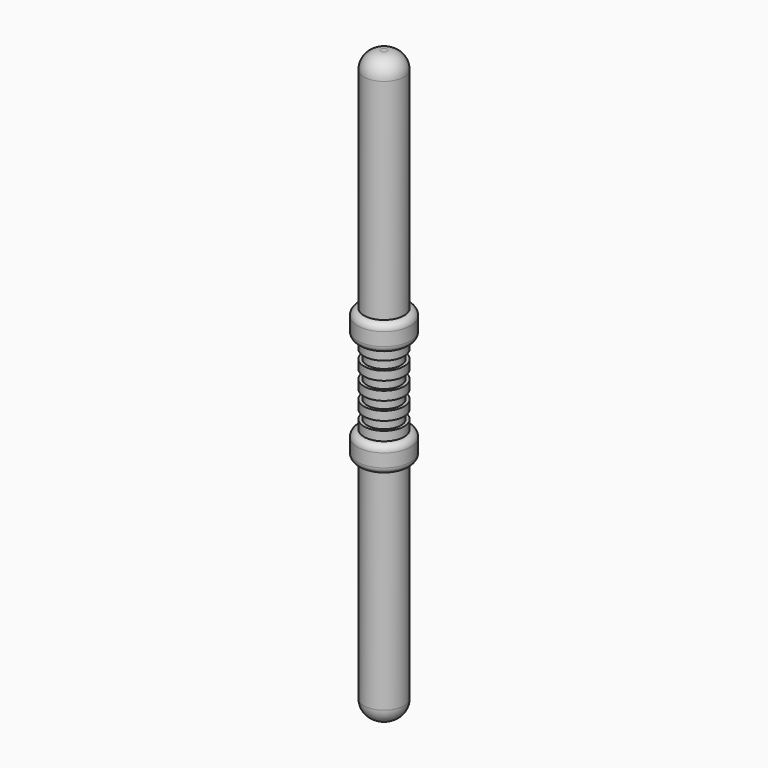
from build123d import *

# Parameters (mm, degrees)
F0_R          = 1.5
F1_DEPTH      = 3
F2_R          = 2
F3_DEPTH      = 2
F4_R          = 1.5
F5_DEPTH      = 17
F6_R          = 1.27
F8_W          = 0.5104065668
F8_H          = 0.6614452832
F10_S5_R      = 1.5
F10_T6_DEPTH  = 5
F10_S11_R     = 1.5
F10_T12_DEPTH = 5
F10_S17_R     = 1.5
F10_T18_DEPTH = 5
F10_S23_R     = 1.5
F10_T24_DEPTH = 5


# Not quite as in the source:
# - a fillet or chamfer that OpenCascade refuses, or shapes differently, is made with other operations: its cross-section is extruded or revolved along the edge and cut away or added


with BuildPart() as f1:
    # F0 (on Top) → F1 (new body, symmetric)
    with BuildSketch(Plane.XY):
        Circle(F0_R)
    extrude(amount=F1_DEPTH, both=True)

    # F2 (on face) → F3 (join)
    with BuildSketch(Plane.XY.offset(3)):
        Circle(F2_R)
    extrude(amount=F3_DEPTH)

    # F4 (on face) → F5 (join)
    with BuildSketch(Plane.XY.offset(5)):
        Circle(F4_R)
    extrude(amount=F5_DEPTH)

    # F6
    f6_edges = [f1.edges().sort_by_distance(p)[0] for p in [
        (-1.5, 0, 22),
    ]]
    fillet(f6_edges, radius=F6_R)

    # F7: F1 across plane


with BuildPart() as f1_1:
    add(f1.part)
    add(f1.part.mirror(Plane.XY))

    # F8 (on Front) → F9 (revolve, cut)
    with BuildSketch(Plane.XZ):
        with Locations((1.5252032834, 1.9843358497)):
            Rectangle(F8_W, F8_H)
        with Locations((1.5252032834, 0.6614452832)):
            Rectangle(F8_W, F8_H)
        with Locations((1.5252032834, -0.6614452832)):
            Rectangle(F8_W, F8_H)
        with Locations((1.5252032834, -1.9843358497)):
            Rectangle(F8_W, F8_H)
    revolve(axis=Axis((0, 0, 0.6306489231), (0, 0, 1)), mode=Mode.SUBTRACT)

    # F10: fillet of radius 0.508 on 4 edges, made by hand


with BuildPart() as f10_tool2:
    # F10_s3 → F10_t4 (revolve)
    with BuildSketch(Plane.XZ):
        with BuildLine():
            ThreePointArc((1.492, 5), (1.8512102448, 4.8512102448), (2, 4.492))
            Line((2, 4.492), (2, 5))
            Line((2, 5), (1.492, 5))
        make_face()
    revolve(axis=Axis((0, 0, 5), (0, 0, 1)))

    # F10_s5 → F10_t6 (cut, symmetric)
    with BuildSketch(Plane.XY.offset(4.6)):
        Circle(F10_S5_R)
    extrude(amount=F10_T6_DEPTH, both=True, mode=Mode.SUBTRACT)


with BuildPart() as f1_2:
    add(f1_1.part)

    # F10_t1: cut F10_tool2
    add(f10_tool2.part, mode=Mode.SUBTRACT)


with BuildPart() as f10_tool8:
    # F10_s9 → F10_t10 (revolve)
    with BuildSketch(Plane.XZ):
        with BuildLine():
            ThreePointArc((2, 3.508), (1.8512102448, 3.1487897552), (1.492, 3))
            Line((1.492, 3), (2, 3))
            Line((2, 3), (2, 3.508))
        make_face()
    revolve(axis=Axis((0, 0, 3), (0, 0, 1)))

    # F10_s11 → F10_t12 (cut, symmetric)
    with BuildSketch(Plane.XY.offset(3.3)):
        Circle(F10_S11_R)
    extrude(amount=F10_T12_DEPTH, both=True, mode=Mode.SUBTRACT)


with BuildPart() as f1_3:
    add(f1_2.part)

    # F10_t7: cut F10_tool8
    add(f10_tool8.part, mode=Mode.SUBTRACT)


with BuildPart() as f10_tool14:
    # F10_s15 → F10_t16 (revolve)
    with BuildSketch(Plane.XZ):
        with BuildLine():
            ThreePointArc((1.492, -3), (1.8512102448, -3.1487897552), (2, -3.508))
            Line((2, -3.508), (2, -3))
            Line((2, -3), (1.492, -3))
        make_face()
    revolve(axis=Axis((0, 0, -3), (0, 0, 1)))

    # F10_s17 → F10_t18 (cut, symmetric)
    with BuildSketch(Plane.XY.offset(-3.4)):
        Circle(F10_S17_R)
    extrude(amount=F10_T18_DEPTH, both=True, mode=Mode.SUBTRACT)


with BuildPart() as f1_4:
    add(f1_3.part)

    # F10_t13: cut F10_tool14
    add(f10_tool14.part, mode=Mode.SUBTRACT)


with BuildPart() as f10_tool20:
    # F10_s21 → F10_t22 (revolve)
    with BuildSketch(Plane.XZ):
        with BuildLine():
            ThreePointArc((2, -4.492), (1.8512102448, -4.8512102448), (1.492, -5))
            Line((1.492, -5), (2, -5))
            Line((2, -5), (2, -4.492))
        make_face()
    revolve(axis=Axis((0, 0, -5), (0, 0, 1)))

    # F10_s23 → F10_t24 (cut, symmetric)
    with BuildSketch(Plane.XY.offset(-4.7)):
        Circle(F10_S23_R)
    extrude(amount=F10_T24_DEPTH, both=True, mode=Mode.SUBTRACT)


with BuildPart() as f1_5:
    add(f1_4.part)

    # F10_t19: cut F10_tool20
    add(f10_tool20.part, mode=Mode.SUBTRACT)


solid = f1_5.part
